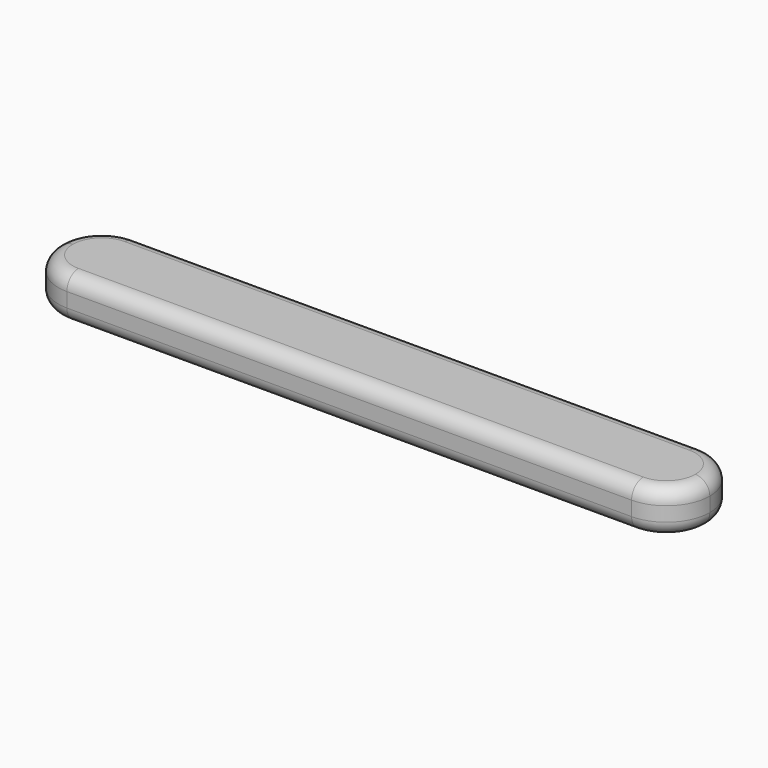
from build123d import *

# Parameters (mm, degrees)
F0_W        = 90
F0_H        = 12
F1_DEPTH    = 6
F2_W        = 5.2
F2_H        = 1.5
F3_DEPTH    = 50
F4_T1_DEPTH = 36
F5_R        = 2


# Not quite as in the source:
# - a fillet or chamfer that OpenCascade refuses, or shapes differently, is made with other operations: its cross-section is extruded or revolved along the edge and cut away or added


with BuildPart() as f1:
    # F0 (on Top) → F1 (new body)
    with BuildSketch(Plane.XY):
        with Locations((-11.5065481514, -2.003862651)):
            Rectangle(F0_W, F0_H)
    extrude(amount=F1_DEPTH)

    # F2 (on face) → F3 (cut)
    with BuildSketch(Plane(origin=(-56.5065481514, 0, 0), x_dir=(0, -1, 0), z_dir=(-1, 0, 0))):
        with Locations((2.003862651, 3)):
            Rectangle(F2_W, F2_H)
    extrude(amount=-F3_DEPTH, mode=Mode.SUBTRACT)

    # F4: fillet of radius 6 on 4 edges, made by hand

    # F4_s2 → F4_t1 (cut)
    with BuildSketch(Plane.XY.offset(-15)):
        with BuildLine():
            ThreePointArc((-56.5065481514, -2.003862651), (-54.7491888385, -6.2465033381), (-50.5065481514, -8.003862651))
            Line((-50.5065481514, -8.003862651), (-56.5065481514, -8.003862651))
            Line((-56.5065481514, -8.003862651), (-56.5065481514, -2.003862651))
        make_face()
        with BuildLine():
            ThreePointArc((-56.5065481514, -2.003862651), (-54.7491888385, 2.2387780361), (-50.5065481514, 3.996137349))
            Line((-50.5065481514, 3.996137349), (-56.5065481514, 3.996137349))
            Line((-56.5065481514, 3.996137349), (-56.5065481514, -2.003862651))
        make_face()
        with BuildLine():
            ThreePointArc((27.4934518486, -8.003862651), (31.7360925357, -6.2465033381), (33.4934518486, -2.003862651))
            Line((33.4934518486, -2.003862651), (33.4934518486, -8.003862651))
            Line((33.4934518486, -8.003862651), (27.4934518486, -8.003862651))
        make_face()
        with BuildLine():
            ThreePointArc((27.4934518486, 3.996137349), (31.7360925357, 2.2387780361), (33.4934518486, -2.003862651))
            Line((33.4934518486, -2.003862651), (33.4934518486, 3.996137349))
            Line((33.4934518486, 3.996137349), (27.4934518486, 3.996137349))
        make_face()
    extrude(amount=F4_T1_DEPTH, mode=Mode.SUBTRACT)

    # F5
    f5_edges = [f1.edges().sort_by_distance(p)[0] for p in [
        (-11.506548, -8.003863, 6),
        (-11.506548, -8.003863, 0),
    ]]
    fillet(f5_edges, radius=F5_R)


solid = f1.part
